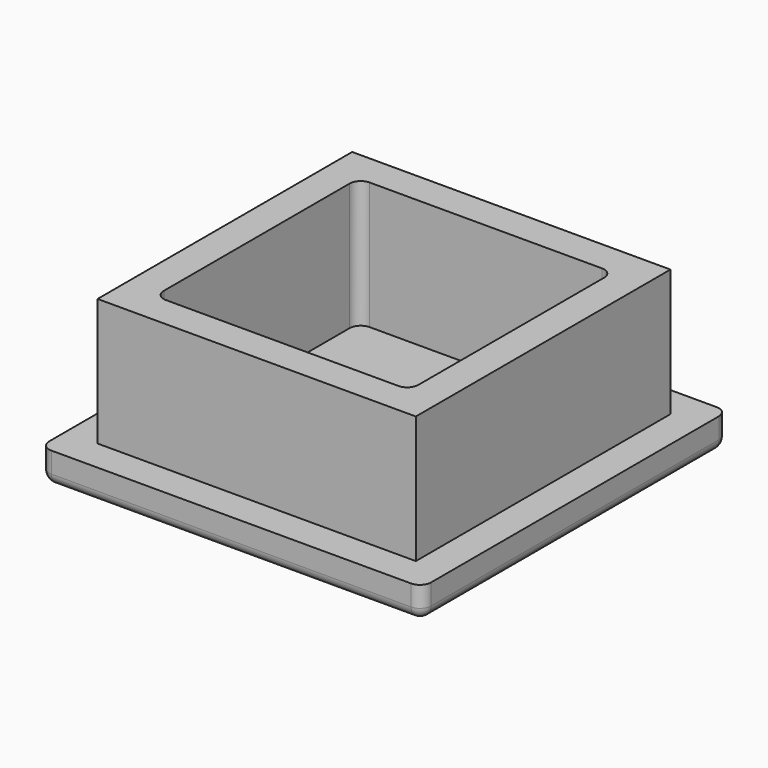
from build123d import *

# Parameters (mm, degrees)
F0_W      = 50.8
F0_H      = 50.8
F1_DEPTH  = 25.4
F2_W      = 40.64
F2_H      = 40.64
F3_DEPTH  = 20.32
F5_W      = 50.8
F5_H      = 50.8
F6_DEPTH  = 25.4
F7_W      = 50.8
F7_H      = 5.08
F8_DEPTH  = 5.08
F10_DEPTH = 5.08
F12_DEPTH = 5.08
F14_DEPTH = 5.08
F15_DEPTH = 25.4
F16_DEPTH = 25.4
F17_R     = 1.778
F18_R     = 1.778
F19_R     = 1.778


# Not quite as in the source:
# - a feature names something its author has since deleted; it is built from what else it names


with BuildPart() as f1:
    # F0 (on Top) → F1 (new body)
    with BuildSketch(Plane.XY):
        with Locations((25.4, 25.4)):
            Rectangle(F0_W, F0_H)
    extrude(amount=F1_DEPTH)

    # F2 (on face) → F3 (cut)
    with BuildSketch(Plane.XY.offset(25.4)):
        with Locations((25.4, 25.4)):
            Rectangle(F2_W, F2_H)
    extrude(amount=-F3_DEPTH, mode=Mode.SUBTRACT)

    # F5 (on face) → F6 (join)
    with BuildSketch(Plane(origin=(0, 0, 0), x_dir=(1, 0, 0), z_dir=(0, 0, -1))):
        with Locations((25.4, -25.4)):
            Rectangle(F5_W, F5_H)
    extrude(amount=F6_DEPTH)

    # F7 (on face) → F8 (join)
    with BuildSketch(Plane(origin=(0, 0, 0), x_dir=(0, -1, 0), z_dir=(-1, 0, 0))):
        with Locations((-25.4, -22.86)):
            Rectangle(F7_W, F7_H)
    extrude(amount=F8_DEPTH)

    # F9 (on face) → F10 (join)
    with BuildSketch(Plane(origin=(0, 50.8, 0), x_dir=(-1, 0, 0), z_dir=(0, 1, 0))):
        Polygon((5.08, -25.4), (5.08, -20.32), (0, -20.32), (-50.8, -20.32), (-50.8, -25.4), align=None)
    extrude(amount=F10_DEPTH)

    # F11 (on face) → F12 (join)
    with BuildSketch(Plane.YZ.offset(50.8)):
        Polygon((55.88, -25.4), (55.88, -20.32), (50.8, -20.32), (0, -20.32), (0, -25.4), align=None)
    extrude(amount=F12_DEPTH)

    # F13 (on face) → F14 (join)
    with BuildSketch(Plane.XZ):
        Polygon((55.88, -25.4), (55.88, -20.32), (50.8, -20.32), (0, -20.32), (-5.08, -20.32), (-5.08, -25.4), align=None)
    extrude(amount=F14_DEPTH)

    # F15 (cut): a face of the model
    f15_faces = [f1.faces().sort_by_distance(p)[0] for p in [
        (25.4, 25.4, 5.08),
    ]]
    extrude(f15_faces, amount=-F15_DEPTH, mode=Mode.SUBTRACT)

    # F16 (cut): a face of the model
    f16_faces = [f1.faces().sort_by_distance(p)[0] for p in [
        (0.7184204897, 25.4, 25.4),
    ]]
    extrude(f16_faces, amount=-F16_DEPTH, mode=Mode.SUBTRACT)

    # F17
    f17_edges = [f1.edges().sort_by_distance(p)[0] for p in [
        (-5.08, -5.08, -22.86),
        (55.88, -5.08, -22.86),
        (55.88, 55.88, -22.86),
        (-5.08, 55.88, -22.86),
    ]]
    fillet(f17_edges, radius=F17_R)

    # F18
    f18_edges = [f1.edges().sort_by_distance(p)[0] for p in [
        (45.72, 45.72, -10.16),
        (5.08, 45.72, -10.16),
        (5.08, 5.08, -10.16),
        (45.72, 5.08, -10.16),
    ]]
    fillet(f18_edges, radius=F18_R)

    # F19
    f19_edges = [f1.edges().sort_by_distance(p)[0] for p in [
        (25.4, -5.08, -25.4),
        (-5.08, 25.4, -25.4),
        (55.88, 25.4, -25.4),
        (25.4, 55.88, -25.4),
        (55.359236, 55.359236, -25.4),
        (-4.559236, 55.359236, -25.4),
        (-4.559236, -4.559236, -25.4),
        (55.359236, -4.559236, -25.4),
    ]]
    fillet(f19_edges, radius=F19_R)


solid = f1.part
